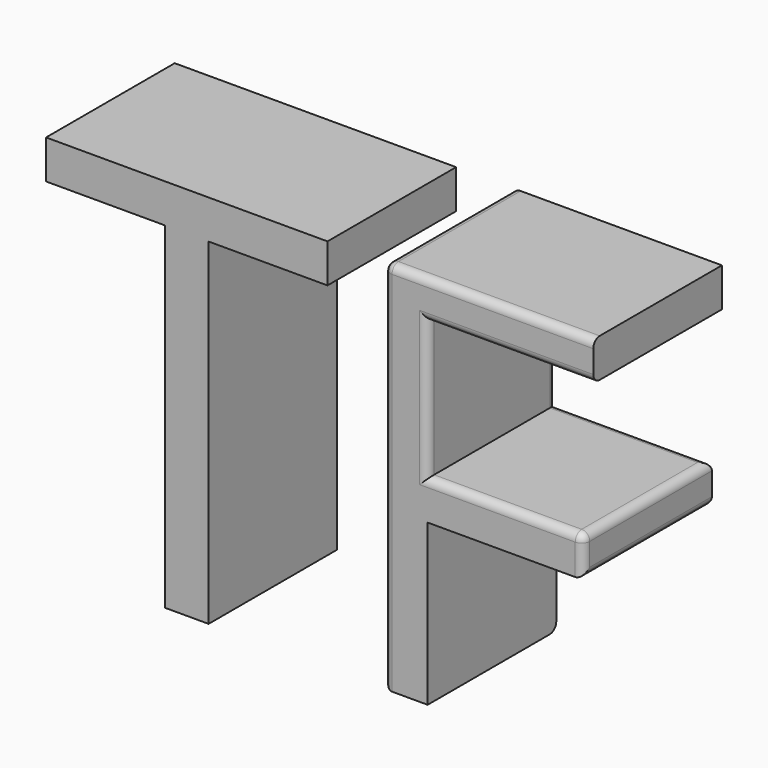
from build123d import *

# Parameters (mm, degrees)
F0_TEXT_SIZE = 83.0774247232
F1_DEPTH     = 25.4
F2_R         = 1.27


# Not quite as in the source:
# - Text() gives the source's letters only with a copy of the font that has no kerning and outlines rounded to 1/6400 em; it was checked with that copy


with BuildPart() as f1:
    # F0 (on Front) → F1 (new body)
    with BuildSketch(Plane.XZ):
        with Locations((54.6964406967, -10.1954042912)):
            Text('TF', F0_TEXT_SIZE, font='Open Sans', text_align=(TextAlign.LEFT, TextAlign.BOTTOM))
    extrude(amount=F1_DEPTH)

    # F2
    f2_edges = [f1.edges().sort_by_distance(p)[0] for p in [
        (125.344704, -25.4, 49.114088),
        (128.791119, -25.4, 42.987128),
        (115.706424, 0, 32.13514),
        (115.706424, -25.4, 32.13514),
        (108.813594, -25.4, 19.459342),
        (127.999287, -25.4, 21.283151),
        (127.999287, 0, 21.283151),
        (140.29215, -12.7, 21.283151),
        (140.29215, -12.7, 15.156191),
        (140.29215, -25.4, 18.219671),
        (127.999287, 0, 15.156191),
        (112.260009, 0, -10.195404),
        (108.813594, -12.7, -10.195404),
        (108.813594, -12.7, 49.114088),
    ]]
    fillet(f2_edges, radius=F2_R)


solid = f1.part
